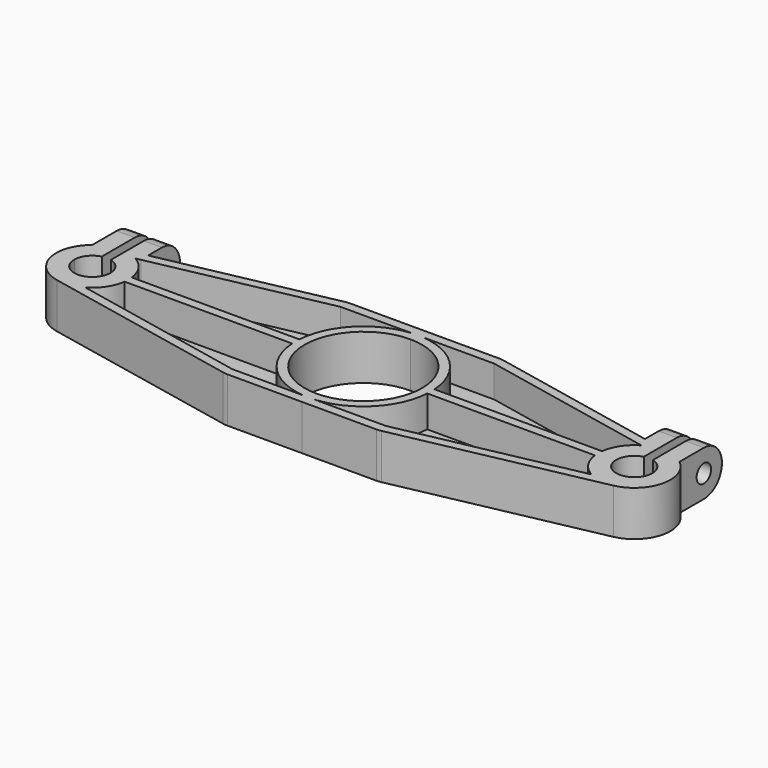
from build123d import *

# Parameters (mm, degrees)
F1_DEPTH = 3
F2_DEPTH = 10
F3_R     = 2
F4_DEPTH = 12
F5_R     = 4.99999


# Not quite as in the source:
# - a fillet or chamfer is up to 0.001 mm smaller than in the source, because OpenCascade refuses the exact size


with BuildPart() as f1:
    # F0 (on Top) → F1 (new body)
    with BuildSketch(Plane.XY):
        Polygon((-59, 8.3724593218), (-55, 9.1941298626), (-55, 18), (-59, 18), align=None)
        with BuildLine():
            Line((-56.0240224388, 6.9420171732), (-55, 7.1523694409))
            Line((-55, 7.1523694409), (-55, 9.1941298626))
            Line((-55, 9.1941298626), (-59, 8.3724593218))
            Line((-59, 8.3724593218), (-59, 7.9372539332))
            ThreePointArc((-59, 7.9372539332), (-57.4627352868, 7.5869814667), (-56.0240224388, 6.9420171732))
        make_face()
        with BuildLine():
            Line((-55, 0), (-55, 6.2449979984))
            ThreePointArc((-55, 6.2449979984), (-55.4985000025, 6.6133575264), (-56.0240224388, 6.9420171732))
            ThreePointArc((-56.0240224388, 6.9420171732), (-57.4627352868, 7.5869814667), (-59, 7.9372539332))
            Line((-59, 7.9372539332), (-59, 3.8729833462))
            ThreePointArc((-59, 3.8729833462), (-56.8377223398, 2.4494897428), (-56, 0))
            Line((-56, 0), (-55, 0))
        make_face()
        with BuildLine():
            ThreePointArc((-61.6097295884, 7.8363748412), (-63.3993016006, 7.2418746626), (-65, 6.2449979984))
            Line((-65, 6.2449979984), (-65, 0))
            Line((-65, 0), (-64, 0))
            ThreePointArc((-64, 0), (-63.1622776602, 2.4494897428), (-61, 3.8729833462))
            Line((-61, 3.8729833462), (-61, 7.9372539332))
            ThreePointArc((-61, 7.9372539332), (-61.3058393006, 7.8927044618), (-61.6097295884, 7.8363748412))
        make_face()
        with BuildLine():
            Line((-65, 18), (-65, 6.2449979984))
            ThreePointArc((-65, 6.2449979984), (-63.3993016006, 7.2418746626), (-61.6097295884, 7.8363748412))
            Line((-61.6097295884, 7.8363748412), (-61, 7.9616240514))
            Line((-61, 7.9616240514), (-61, 18))
            Line((-61, 18), (-65, 18))
        make_face()
        with BuildLine():
            ThreePointArc((-61.6097295884, -7.8363748412), (-58.7351872562, -7.8993828065), (-56.0240224388, -6.9420171732))
            ThreePointArc((-56.0240224388, -6.9420171732), (-53.3435622754, -4.4375485145), (-52.0627460668, -1))
            ThreePointArc((-52.0627460668, -1), (-52.0157019261, -0.5009833003), (-52, 0))
            ThreePointArc((-52, 0), (-52.0157019261, 0.5009833003), (-52.0627460668, 1))
            ThreePointArc((-52.0627460668, 1), (-53.0199831065, 3.9088827261), (-55, 6.2449979984))
            Line((-55, 6.2449979984), (-55, 0))
            Line((-55, 0), (-56, 0))
            ThreePointArc((-56, 0), (-60, -4), (-64, 0))
            Line((-64, 0), (-65, 0))
            Line((-65, 0), (-65, 6.2449979984))
            ThreePointArc((-65, 6.2449979984), (-67.7777500969, -1.8725927026), (-61.6097295884, -7.8363748412))
        make_face()
        with BuildLine():
            Line((-56.0240224388, -6.9420171732), (-17, -14.9582395784))
            Line((-17, -14.9582395784), (-17, -1))
            Line((-17, -1), (-52.0627460668, -1))
            ThreePointArc((-52.0627460668, -1), (-53.3435622754, -4.4375485145), (-56.0240224388, -6.9420171732))
        make_face()
        with BuildLine():
            Line((-17, 1), (-17, 14.9582395784))
            Line((-17, 14.9582395784), (-55, 7.1523694409))
            Line((-55, 7.1523694409), (-55, 6.2449979984))
            ThreePointArc((-55, 6.2449979984), (-53.0199831065, 3.9088827261), (-52.0627460668, 1))
            Line((-52.0627460668, 1), (-17, 1))
        make_face()
        Polygon((-55, 7.1523694409), (-17, 14.9582395784), (-17, 17), (-55, 9.1941298626), align=None)
        with BuildLine():
            Line((-17, -1), (-17, 1))
            Line((-17, 1), (-52.0627460668, 1))
            ThreePointArc((-52.0627460668, 1), (-52.0157019261, 0.5009833003), (-52, 0))
            ThreePointArc((-52, 0), (-52.0157019261, -0.5009833003), (-52.0627460668, -1))
            Line((-52.0627460668, -1), (-17, -1))
        make_face()
        with BuildLine():
            Line((-17, -17), (-17, -14.9582395784))
            Line((-17, -14.9582395784), (-56.0240224388, -6.9420171732))
            ThreePointArc((-56.0240224388, -6.9420171732), (-58.7351872562, -7.8993828065), (-61.6097295884, -7.8363748412))
            Line((-61.6097295884, -7.8363748412), (-17, -17))
        make_face()
        with BuildLine():
            Line((0, -17), (0, -15))
            ThreePointArc((0, -15), (-0.5596455685, -14.9895562589), (-1.1185118312, -14.9582395784))
            Line((-1.1185118312, -14.9582395784), (-17, -14.9582395784))
            Line((-17, -14.9582395784), (-17, -17))
            Line((-17, -17), (0, -17))
        make_face()
        with BuildLine():
            Line((0, -15), (0, -14.9582395784))
            Line((0, -14.9582395784), (-1.1185118312, -14.9582395784))
            ThreePointArc((-1.1185118312, -14.9582395784), (-0.5596455685, -14.9895562589), (0, -15))
        make_face()
        with BuildLine():
            Line((-17, -14.9582395784), (-1.1185118312, -14.9582395784))
            ThreePointArc((-1.1185118312, -14.9582395784), (-10.6485236686, -10.5645134142), (-14.9666295471, -1))
            Line((-14.9666295471, -1), (-17, -1))
            Line((-17, -1), (-17, -14.9582395784))
        make_face()
        with BuildLine():
            ThreePointArc((0, -13), (-13, 0), (0, 13))
            Line((0, 13), (0, 14.9582395784))
            Line((0, 14.9582395784), (-1.1185118312, 14.9582395784))
            ThreePointArc((-1.1185118312, 14.9582395784), (-10.6485236686, 10.5645134142), (-14.9666295471, 1))
            ThreePointArc((-14.9666295471, 1), (-15, 0), (-14.9666295471, -1))
            ThreePointArc((-14.9666295471, -1), (-10.6485236686, -10.5645134142), (-1.1185118312, -14.9582395784))
            Line((-1.1185118312, -14.9582395784), (0, -14.9582395784))
            Line((0, -14.9582395784), (0, -13))
        make_face()
        with BuildLine():
            ThreePointArc((-14.9666295471, -1), (-15, 0), (-14.9666295471, 1))
            Line((-14.9666295471, 1), (-17, 1))
            Line((-17, 1), (-17, -1))
            Line((-17, -1), (-14.9666295471, -1))
        make_face()
        with BuildLine():
            ThreePointArc((-14.9666295471, 1), (-10.6485236686, 10.5645134142), (-1.1185118312, 14.9582395784))
            Line((-1.1185118312, 14.9582395784), (-17, 14.9582395784))
            Line((-17, 14.9582395784), (-17, 1))
            Line((-17, 1), (-14.9666295471, 1))
        make_face()
        with BuildLine():
            ThreePointArc((-1.1185118312, 14.9582395784), (-0.5596455685, 14.9895562589), (0, 15))
            Line((0, 15), (0, 17))
            Line((0, 17), (-17, 17))
            Line((-17, 17), (-17, 14.9582395784))
            Line((-17, 14.9582395784), (-1.1185118312, 14.9582395784))
        make_face()
        with BuildLine():
            Line((-1.1185118312, 14.9582395784), (0, 14.9582395784))
            Line((0, 14.9582395784), (0, 15))
            ThreePointArc((0, 15), (-0.5596455685, 14.9895562589), (-1.1185118312, 14.9582395784))
        make_face()
        with BuildLine():
            Line((-55, 6.2449979984), (-55, 7.1523694409))
            Line((-55, 7.1523694409), (-56.0240224388, 6.9420171732))
            ThreePointArc((-56.0240224388, 6.9420171732), (-55.4985000025, 6.6133575264), (-55, 6.2449979984))
        make_face()
    extrude(amount=F1_DEPTH)

    # F0 (on Top) → F2 (join)
    with BuildSketch(Plane.XY):
        with BuildLine():
            Line((0, -17), (0, -15))
            ThreePointArc((0, -15), (-0.5596455685, -14.9895562589), (-1.1185118312, -14.9582395784))
            Line((-1.1185118312, -14.9582395784), (-17, -14.9582395784))
            Line((-17, -14.9582395784), (-17, -17))
            Line((-17, -17), (0, -17))
        make_face()
        with BuildLine():
            Line((0, -15), (0, -14.9582395784))
            Line((0, -14.9582395784), (-1.1185118312, -14.9582395784))
            ThreePointArc((-1.1185118312, -14.9582395784), (-0.5596455685, -14.9895562589), (0, -15))
        make_face()
        with BuildLine():
            Line((-17, -17), (-17, -14.9582395784))
            Line((-17, -14.9582395784), (-56.0240224388, -6.9420171732))
            ThreePointArc((-56.0240224388, -6.9420171732), (-58.7351872562, -7.8993828065), (-61.6097295884, -7.8363748412))
            Line((-61.6097295884, -7.8363748412), (-17, -17))
        make_face()
        with BuildLine():
            ThreePointArc((0, -13), (-13, 0), (0, 13))
            Line((0, 13), (0, 14.9582395784))
            Line((0, 14.9582395784), (-1.1185118312, 14.9582395784))
            ThreePointArc((-1.1185118312, 14.9582395784), (-10.6485236686, 10.5645134142), (-14.9666295471, 1))
            ThreePointArc((-14.9666295471, 1), (-15, 0), (-14.9666295471, -1))
            ThreePointArc((-14.9666295471, -1), (-10.6485236686, -10.5645134142), (-1.1185118312, -14.9582395784))
            Line((-1.1185118312, -14.9582395784), (0, -14.9582395784))
            Line((0, -14.9582395784), (0, -13))
        make_face()
        with BuildLine():
            ThreePointArc((-1.1185118312, 14.9582395784), (-0.5596455685, 14.9895562589), (0, 15))
            Line((0, 15), (0, 17))
            Line((0, 17), (-17, 17))
            Line((-17, 17), (-17, 14.9582395784))
            Line((-17, 14.9582395784), (-1.1185118312, 14.9582395784))
        make_face()
        with BuildLine():
            Line((-1.1185118312, 14.9582395784), (0, 14.9582395784))
            Line((0, 14.9582395784), (0, 15))
            ThreePointArc((0, 15), (-0.5596455685, 14.9895562589), (-1.1185118312, 14.9582395784))
        make_face()
        Polygon((-55, 7.1523694409), (-17, 14.9582395784), (-17, 17), (-55, 9.1941298626), align=None)
        with BuildLine():
            Line((-56.0240224388, 6.9420171732), (-55, 7.1523694409))
            Line((-55, 7.1523694409), (-55, 9.1941298626))
            Line((-55, 9.1941298626), (-59, 8.3724593218))
            Line((-59, 8.3724593218), (-59, 7.9372539332))
            ThreePointArc((-59, 7.9372539332), (-57.4627352868, 7.5869814667), (-56.0240224388, 6.9420171732))
        make_face()
        with BuildLine():
            ThreePointArc((-61.6097295884, -7.8363748412), (-58.7351872562, -7.8993828065), (-56.0240224388, -6.9420171732))
            ThreePointArc((-56.0240224388, -6.9420171732), (-53.3435622754, -4.4375485145), (-52.0627460668, -1))
            ThreePointArc((-52.0627460668, -1), (-52.0157019261, -0.5009833003), (-52, 0))
            ThreePointArc((-52, 0), (-52.0157019261, 0.5009833003), (-52.0627460668, 1))
            ThreePointArc((-52.0627460668, 1), (-53.0199831065, 3.9088827261), (-55, 6.2449979984))
            Line((-55, 6.2449979984), (-55, 0))
            Line((-55, 0), (-56, 0))
            ThreePointArc((-56, 0), (-60, -4), (-64, 0))
            Line((-64, 0), (-65, 0))
            Line((-65, 0), (-65, 6.2449979984))
            ThreePointArc((-65, 6.2449979984), (-67.7777500969, -1.8725927026), (-61.6097295884, -7.8363748412))
        make_face()
        with BuildLine():
            Line((-55, 0), (-55, 6.2449979984))
            ThreePointArc((-55, 6.2449979984), (-55.4985000025, 6.6133575264), (-56.0240224388, 6.9420171732))
            ThreePointArc((-56.0240224388, 6.9420171732), (-57.4627352868, 7.5869814667), (-59, 7.9372539332))
            Line((-59, 7.9372539332), (-59, 3.8729833462))
            ThreePointArc((-59, 3.8729833462), (-56.8377223398, 2.4494897428), (-56, 0))
            Line((-56, 0), (-55, 0))
        make_face()
        with BuildLine():
            ThreePointArc((-61.6097295884, 7.8363748412), (-63.3993016006, 7.2418746626), (-65, 6.2449979984))
            Line((-65, 6.2449979984), (-65, 0))
            Line((-65, 0), (-64, 0))
            ThreePointArc((-64, 0), (-63.1622776602, 2.4494897428), (-61, 3.8729833462))
            Line((-61, 3.8729833462), (-61, 7.9372539332))
            ThreePointArc((-61, 7.9372539332), (-61.3058393006, 7.8927044618), (-61.6097295884, 7.8363748412))
        make_face()
        with BuildLine():
            Line((-65, 18), (-65, 6.2449979984))
            ThreePointArc((-65, 6.2449979984), (-63.3993016006, 7.2418746626), (-61.6097295884, 7.8363748412))
            Line((-61.6097295884, 7.8363748412), (-61, 7.9616240514))
            Line((-61, 7.9616240514), (-61, 18))
            Line((-61, 18), (-65, 18))
        make_face()
        Polygon((-59, 8.3724593218), (-55, 9.1941298626), (-55, 18), (-59, 18), align=None)
        with BuildLine():
            Line((-17, -1), (-17, 1))
            Line((-17, 1), (-52.0627460668, 1))
            ThreePointArc((-52.0627460668, 1), (-52.0157019261, 0.5009833003), (-52, 0))
            ThreePointArc((-52, 0), (-52.0157019261, -0.5009833003), (-52.0627460668, -1))
            Line((-52.0627460668, -1), (-17, -1))
        make_face()
        with BuildLine():
            ThreePointArc((-14.9666295471, -1), (-15, 0), (-14.9666295471, 1))
            Line((-14.9666295471, 1), (-17, 1))
            Line((-17, 1), (-17, -1))
            Line((-17, -1), (-14.9666295471, -1))
        make_face()
        with BuildLine():
            Line((-61, 7.9372539332), (-61, 7.9616240514))
            Line((-61, 7.9616240514), (-61.6097295884, 7.8363748412))
            ThreePointArc((-61.6097295884, 7.8363748412), (-61.3058393006, 7.8927044618), (-61, 7.9372539332))
        make_face()
    extrude(amount=F2_DEPTH)

    # F3 (on face) → F4 (cut)
    with BuildSketch(Plane(origin=(-65, 0, 0), x_dir=(0, -1, 0), z_dir=(-1, 0, 0))):
        with Locations((-13, 5)):
            Circle(F3_R)
    extrude(amount=-F4_DEPTH, mode=Mode.SUBTRACT)

    # F5 (radius 5 in the source; OpenCascade refuses exactly that, so slightly less here)
    f5_edges = [f1.edges().sort_by_distance(p)[0] for p in [
        (-63, 18, 0),
        (-57, 18, 0),
        (-57, 18, 10),
        (-63, 18, 10),
        (-17, 17, 5),
        (-17, -17, 5),
    ]]
    fillet(f5_edges, radius=F5_R)

    # F6: F1 across face


with BuildPart() as f1_1:
    add(f1.part)
    add(f1.part.mirror(Plane(origin=(0, -15, 5), x_dir=(0, 1, 0), z_dir=(1, 0, 0))))


solid = f1_1.part
